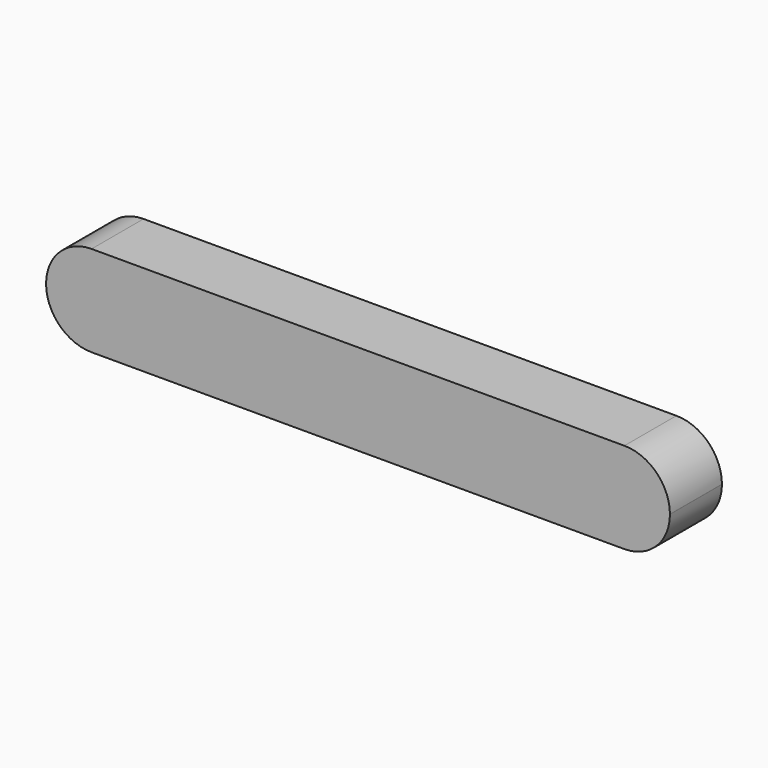
from build123d import *

# Parameters (mm, degrees)
F1_DEPTH = 15.875


# Not quite as in the source:
# - ends of sketch curves that miss each other by under 0.0002 mm in the source are joined


with BuildPart() as f1:
    # F0 (on Front) → F1 (new body)
    with BuildSketch(Plane.XZ):
        with BuildLine():
            Line((99.3167190849, 6.0181862739), (-30.8455809151, 6.0181862739))
            ThreePointArc((-30.8455809151, 6.0181862739), (-38.6988136123, 2.7678992228), (-41.958073658, -5.0816137344))
            Line((-41.958073658, -5.0816137344), (-41.9580809151, -5.0943137261))
            ThreePointArc((-41.9580809151, -5.0943137261), (-38.6950938699, -12.9528069326), (-30.8328809151, -16.2068137261))
            Line((-30.8328809151, -16.2068137261), (99.3167190849, -16.2068137261))
            ThreePointArc((99.3167190849, -16.2068137261), (107.1744380827, -12.957293201), (110.4418900895, -5.1070136599))
            Line((110.4418900895, -5.1070136599), (110.4419190849, -5.0816137261))
            ThreePointArc((110.4419190849, -5.0816137261), (107.1744380827, 2.7686657488), (99.3167190849, 6.0181862739))
        make_face()
    extrude(amount=F1_DEPTH)


solid = f1.part
